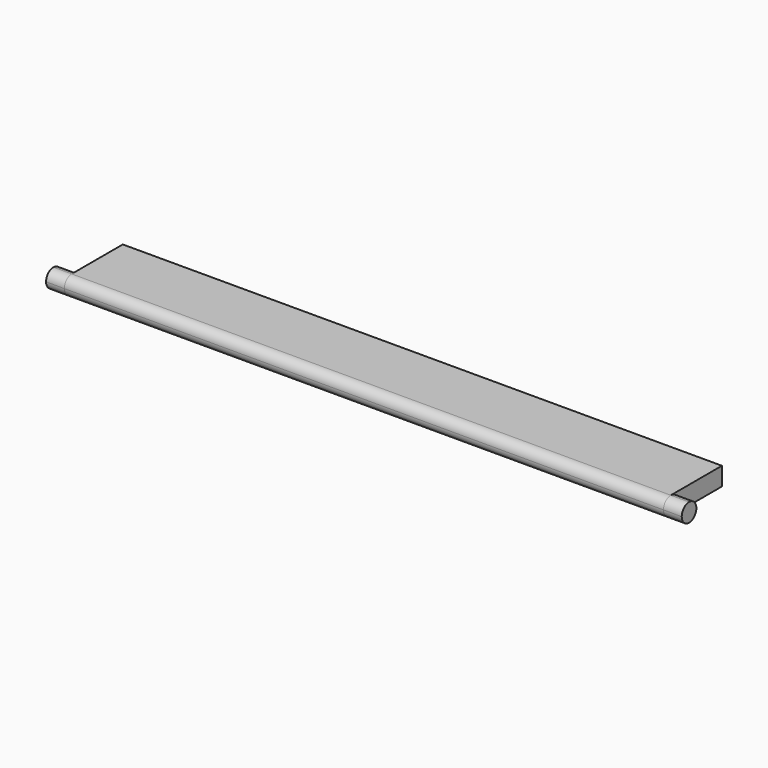
from build123d import *
from build123d import SkipClean  # not in build123d's __all__

# Parameters (mm, degrees)
F0_W     = 52.07
F0_H     = 6.35
F1_DEPTH = 1.5875
F3_DEPTH = 1.5875
F5_DEPTH = 1.5875
F6_DEPTH = 52.07


with BuildPart() as f1:
    # F0 (on Top) → F1 (new body)
    with BuildSketch(Plane.XY):
        with Locations((12.0531544089, -15.5635510429)):
            Rectangle(F0_W, F0_H)
    extrude(amount=F1_DEPTH)

    # F2 (on face) → F3 (join)
    with BuildSketch(Plane(origin=(-13.9818455911, 0, 0), x_dir=(0, -1, 0), z_dir=(-1, 0, 0))):
        with BuildLine():
            ThreePointArc((17.9448010429, 0), (18.5060670505, 0.2324839924), (18.7385510429, 0.79375))
            ThreePointArc((18.7385510429, 0.79375), (18.5060670505, 1.3550160076), (17.9448010429, 1.5875))
            ThreePointArc((17.9448010429, 1.5875), (17.1510510429, 0.79375), (17.9448010429, 0))
        make_face()
    extrude(amount=F3_DEPTH)

    # F4 (on face) → F5 (join)
    with BuildSketch(Plane.YZ.offset(38.0881544089)):
        with BuildLine():
            ThreePointArc((-17.9448010429, 0), (-17.3835350353, 0.2324839924), (-17.1510510429, 0.79375))
            ThreePointArc((-17.1510510429, 0.79375), (-17.3835350353, 1.3550160076), (-17.9448010429, 1.5875))
            ThreePointArc((-17.9448010429, 1.5875), (-18.5060670505, 1.3550160076), (-18.7385510429, 0.79375))
            ThreePointArc((-18.7385510429, 0.79375), (-18.5060670505, 0.2324839924), (-17.9448010429, 0))
        make_face()
    extrude(amount=F5_DEPTH)

    # F6 (cut): faces of the model
    f6_faces = [f1.faces().sort_by_distance(p)[0] for p in [
        (38.0881544089, -18.5612527414, 1.4102016985),
        (38.0881544089, -18.5612527414, 0.1772983015),
    ]]
    with SkipClean():  # cleaning this boolean's faces spoils the solid; the shape is the same uncleaned
        extrude(f6_faces, amount=-F6_DEPTH, mode=Mode.SUBTRACT)


solid = f1.part
